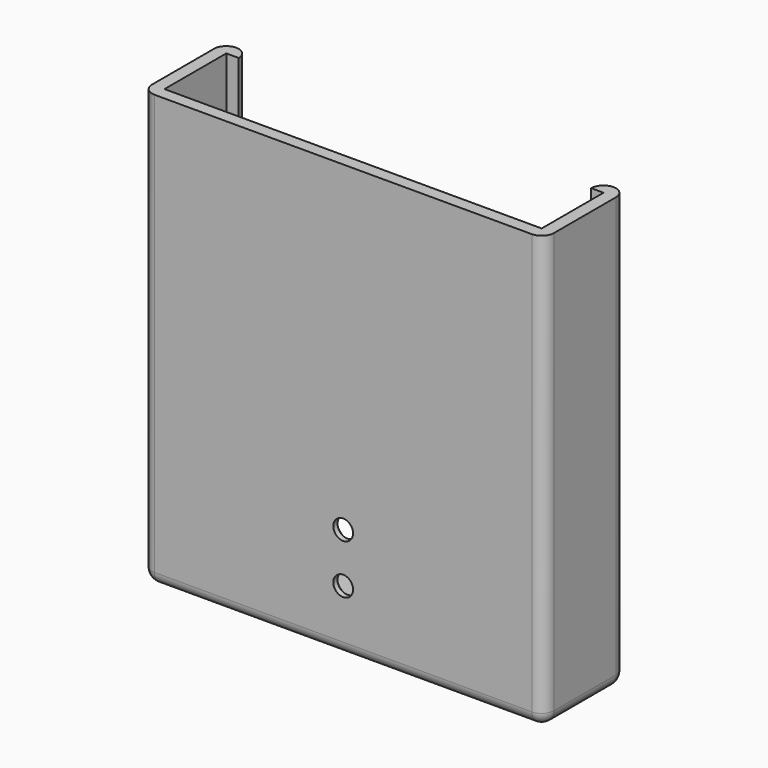
from build123d import *

# Parameters (mm, degrees)
F0_DEPTH       = 70
F1_W           = 65
F1_H           = 16.5
F8_DEPTH       = 2
F2_T1_DEPTH    = 12.5
F2_T3_DEPTH    = 73
F2_T5_DEPTH    = 57
F2_T7_DEPTH    = 61
F2_S11_W       = 2.04
F2_S11_H       = 2.04
F2_T12_DEPTH   = 2.04
F2_S17_W       = 2.04
F2_S17_H       = 2.04
F2_T18_DEPTH   = 2.04
F2_S23_W       = 2.04
F2_S23_H       = 2.04
F2_T24_DEPTH   = 2.04
F2_S29_W       = 2.04
F2_S29_H       = 2.04
F2_T30_DEPTH   = 2.04
F2_T37_DEPTH   = 73
F2_T42_DEPTH   = 62
F2_T50_DEPTH   = 62
F2_T55_DEPTH   = 73
F2_T62_DEPTH   = 17.5
F2_T67_DEPTH   = 17.5
F5_D           = 3.2
F5_CSINK_D     = 5.5
F5_CSINK_ANGLE = 90
F6_D           = 3.2
F6_CSINK_D     = 5.5
F6_CSINK_ANGLE = 90


# Not quite as in the source:
# - a fillet or chamfer that OpenCascade refuses, or shapes differently, is made with other operations: its cross-section is extruded or revolved along the edge and cut away or added
# - a feature names something its author has since deleted; it is built from what else it names


with BuildPart() as f0:
    # F7 (on Top) → F0 (new body)
    with BuildSketch(Plane.XY):
        Polygon((-32.5, 16.5), (-32.5, 0), (32.5, 0), (32.5, 16.5), (28.5, 16.5), (28.5, 14.5), (30.5, 14.5), (30.5, 2), (-30.5, 2), (-30.5, 14.5), (-28.5, 14.5), (-28.5, 16.5), align=None)
    extrude(amount=F0_DEPTH)

    # F1 (on face) → F8 (join)
    with BuildSketch(Plane(origin=(0, 0, 0), x_dir=(1, 0, 0), z_dir=(0, 0, -1))):
        with Locations((0, -8.25)):
            Rectangle(F1_W, F1_H)
    extrude(amount=-F8_DEPTH)

    # F2: fillet of radius 2 on 13 edges, made by hand

    # F2_s2 → F2_t1 (cut)
    with BuildSketch(Plane.XZ.offset(-14.5)):
        with BuildLine():
            ThreePointArc((32.5, 2), (31.9142135624, 0.5857864376), (30.5, 0))
            Line((30.5, 0), (32.5, 0))
            Line((32.5, 0), (32.5, 2))
        make_face()
        with BuildLine():
            ThreePointArc((-32.5, 2), (-31.9142135624, 0.5857864376), (-30.5, 0))
            Line((-30.5, 0), (-32.5, 0))
            Line((-32.5, 0), (-32.5, 2))
        make_face()
    extrude(amount=F2_T1_DEPTH, mode=Mode.SUBTRACT)

    # F2_s4 → F2_t3 (cut)
    with BuildSketch(Plane.XY.offset(2)):
        with BuildLine():
            ThreePointArc((-32.5, 2), (-31.9142135624, 0.5857864376), (-30.5, 0))
            Line((-30.5, 0), (-32.5, 0))
            Line((-32.5, 0), (-32.5, 2))
        make_face()
        with BuildLine():
            ThreePointArc((30.5, 0), (31.9142135624, 0.5857864376), (32.5, 2))
            Line((32.5, 2), (32.5, 0))
            Line((32.5, 0), (30.5, 0))
        make_face()
        with BuildLine():
            ThreePointArc((-32.5, 14.5), (-31.9142135624, 15.9142135624), (-30.5, 16.5))
            Line((-30.5, 16.5), (-32.5, 16.5))
            Line((-32.5, 16.5), (-32.5, 14.5))
        make_face()
        with BuildLine():
            ThreePointArc((32.5, 14.5), (31.9142135624, 15.9142135624), (30.5, 16.5))
            Line((30.5, 16.5), (32.5, 16.5))
            Line((32.5, 16.5), (32.5, 14.5))
        make_face()
        with BuildLine():
            ThreePointArc((-28.5, 14.5), (-29.0857864376, 15.9142135624), (-30.5, 16.5))
            Line((-30.5, 16.5), (-28.5, 16.5))
            Line((-28.5, 16.5), (-28.5, 14.5))
        make_face()
        with BuildLine():
            ThreePointArc((28.5, 14.5), (29.0857864376, 15.9142135624), (30.5, 16.5))
            Line((30.5, 16.5), (28.5, 16.5))
            Line((28.5, 16.5), (28.5, 14.5))
        make_face()
    extrude(amount=F2_T3_DEPTH, mode=Mode.SUBTRACT)

    # F2_s6 → F2_t5 (cut)
    with BuildSketch(Plane.YZ.offset(-28.5)):
        with BuildLine():
            ThreePointArc((14.5, 2), (15.9142135624, 1.4142135624), (16.5, 0))
            Line((16.5, 0), (16.5, 2))
            Line((16.5, 2), (14.5, 2))
        make_face()
    extrude(amount=F2_T5_DEPTH, mode=Mode.SUBTRACT)

    # F2_s8 → F2_t7 (cut)
    with BuildSketch(Plane.YZ.offset(-30.5)):
        with BuildLine():
            ThreePointArc((0, 2), (0.5857864376, 0.5857864376), (2, 0))
            Line((2, 0), (0, 0))
            Line((0, 0), (0, 2))
        make_face()
        with BuildLine():
            ThreePointArc((16.5, 2), (15.9142135624, 0.5857864376), (14.5, 0))
            Line((14.5, 0), (16.5, 0))
            Line((16.5, 0), (16.5, 2))
        make_face()
    extrude(amount=F2_T7_DEPTH, mode=Mode.SUBTRACT)


with BuildPart() as f2_tool10:
    # F2_s11 → F2_t12 (new body)
    with BuildSketch(Plane.XZ.offset(-2)):
        with Locations((31.52, 0.98)):
            Rectangle(F2_S11_W, F2_S11_H)
    extrude(amount=F2_T12_DEPTH)

    # F2_s13 → F2_t14 (revolve, cut)
    with BuildSketch(Plane(origin=(30.5, 2, 2), x_dir=(-0.7071067812, 0, 0.7071067812), z_dir=(0.7071067812, 0, 0.7071067812))):
        with BuildLine():
            ThreePointArc((0, -2), (2, 0), (0, 2))
            Line((0, 2), (0, -2))
        make_face()
    revolve(axis=Axis((30.5, 2, 2), (0, -1, 0)), mode=Mode.SUBTRACT)


with BuildPart() as f0_1:
    add(f0.part)

    # F2_t9: cut F2_tool10
    add(f2_tool10.part, mode=Mode.SUBTRACT)


with BuildPart() as f2_tool16:
    # F2_s17 → F2_t18 (new body)
    with BuildSketch(Plane.YZ.offset(30.5)):
        with Locations((15.52, 0.98)):
            Rectangle(F2_S17_W, F2_S17_H)
    extrude(amount=F2_T18_DEPTH)

    # F2_s19 → F2_t20 (revolve, cut)
    with BuildSketch(Plane(origin=(30.5, 14.5, 2), x_dir=(0, -0.7071067812, 0.7071067812), z_dir=(0, 0.7071067812, 0.7071067812))):
        with BuildLine():
            ThreePointArc((0, -2), (2, 0), (0, 2))
            Line((0, 2), (0, -2))
        make_face()
    revolve(axis=Axis((30.5, 14.5, 2), (1, 0, 0)), mode=Mode.SUBTRACT)


with BuildPart() as f0_2:
    add(f0_1.part)

    # F2_t15: cut F2_tool16
    add(f2_tool16.part, mode=Mode.SUBTRACT)


with BuildPart() as f2_tool22:
    # F2_s23 → F2_t24 (new body)
    with BuildSketch(Plane.YZ.offset(-30.5)):
        with Locations((15.52, 0.98)):
            Rectangle(F2_S23_W, F2_S23_H)
    extrude(amount=-F2_T24_DEPTH)

    # F2_s25 → F2_t26 (revolve, cut)
    with BuildSketch(Plane(origin=(-30.5, 14.5, 2), x_dir=(0, -0.7071067812, 0.7071067812), z_dir=(0, -0.7071067812, -0.7071067812))):
        with BuildLine():
            ThreePointArc((0, -2), (2, 0), (0, 2))
            Line((0, 2), (0, -2))
        make_face()
    revolve(axis=Axis((-30.5, 14.5, 2), (-1, 0, 0)), mode=Mode.SUBTRACT)


with BuildPart() as f0_3:
    add(f0_2.part)

    # F2_t21: cut F2_tool22
    add(f2_tool22.part, mode=Mode.SUBTRACT)


with BuildPart() as f2_tool28:
    # F2_s29 → F2_t30 (new body)
    with BuildSketch(Plane.YZ.offset(-30.5)):
        with Locations((0.98, 0.98)):
            Rectangle(F2_S29_W, F2_S29_H)
    extrude(amount=-F2_T30_DEPTH)

    # F2_s31 → F2_t32 (revolve, cut)
    with BuildSketch(Plane(origin=(-30.5, 2, 2), x_dir=(0, 0.7071067812, 0.7071067812), z_dir=(0, -0.7071067812, 0.7071067812))):
        with BuildLine():
            ThreePointArc((0, -2), (2, 0), (0, 2))
            Line((0, 2), (0, -2))
        make_face()
    revolve(axis=Axis((-30.5, 2, 2), (-1, 0, 0)), mode=Mode.SUBTRACT)


with BuildPart() as f0_4:
    add(f0_3.part)

    # F2_t27: cut F2_tool28
    add(f2_tool28.part, mode=Mode.SUBTRACT)


with BuildPart() as f2_tool35:
    # F2_s36 → F2_t37 (new body)
    with BuildSketch(Plane.XY.offset(-3)):
        with BuildLine():
            ThreePointArc((-28.5, 14.5), (-29.0857864376, 15.9142135624), (-30.5, 16.5))
            Line((-30.5, 16.5), (-28.5, 16.5))
            Line((-28.5, 16.5), (-28.5, 14.5))
        make_face()
    extrude(amount=F2_T37_DEPTH)

    split(bisect_by=Plane.XY.offset(2), keep=Keep.BOTTOM)

    split(bisect_by=Plane.XY, keep=Keep.TOP)


with BuildPart() as f2_tool40:
    # F2_s41 → F2_t42 (new body)
    with BuildSketch(Plane.YZ.offset(-33.5)):
        with BuildLine():
            ThreePointArc((14.5, 2), (15.9142135624, 1.4142135624), (16.5, 0))
            Line((16.5, 0), (16.5, 2))
            Line((16.5, 2), (14.5, 2))
        make_face()
    extrude(amount=F2_T42_DEPTH)

    split(bisect_by=Plane.YZ.offset(-28.5), keep=Keep.BOTTOM)

    split(bisect_by=Plane.YZ.offset(-30.5), keep=Keep.TOP)


with BuildPart() as f2_tool35_1:
    add(f2_tool35.part)

    # F2_t45: intersect F2_tool40
    add(f2_tool40.part, mode=Mode.INTERSECT)


with BuildPart() as f0_5:
    add(f0_4.part)

    # F2_t33: cut F2_tool35
    add(f2_tool35_1.part, mode=Mode.SUBTRACT)


with BuildPart() as f2_tool48:
    # F2_s49 → F2_t50 (new body)
    with BuildSketch(Plane.YZ.offset(-28.5)):
        with BuildLine():
            ThreePointArc((14.5, 2), (15.9142135624, 1.4142135624), (16.5, 0))
            Line((16.5, 0), (16.5, 2))
            Line((16.5, 2), (14.5, 2))
        make_face()
    extrude(amount=F2_T50_DEPTH)

    split(bisect_by=Plane.YZ.offset(30.5), keep=Keep.BOTTOM)

    split(bisect_by=Plane.YZ.offset(28.5), keep=Keep.TOP)


with BuildPart() as f2_tool53:
    # F2_s54 → F2_t55 (new body)
    with BuildSketch(Plane.XY.offset(-3)):
        with BuildLine():
            ThreePointArc((28.5, 14.5), (29.0857864376, 15.9142135624), (30.5, 16.5))
            Line((30.5, 16.5), (28.5, 16.5))
            Line((28.5, 16.5), (28.5, 14.5))
        make_face()
    extrude(amount=F2_T55_DEPTH)

    split(bisect_by=Plane.XY.offset(2), keep=Keep.BOTTOM)

    split(bisect_by=Plane.XY, keep=Keep.TOP)


with BuildPart() as f2_tool48_1:
    add(f2_tool48.part)

    # F2_t58: intersect F2_tool53
    add(f2_tool53.part, mode=Mode.INTERSECT)


with BuildPart() as f0_6:
    add(f0_5.part)

    # F2_t46: cut F2_tool48
    add(f2_tool48_1.part, mode=Mode.SUBTRACT)


with BuildPart() as f2_tool60:
    # F2_s61 → F2_t62 (new body)
    with BuildSketch(Plane.XZ.offset(3)):
        with BuildLine():
            ThreePointArc((30.5, 4), (29.9142135624, 2.5857864376), (28.5, 2))
            Line((28.5, 2), (30.5, 2))
            Line((30.5, 2), (30.5, 4))
        make_face()
    extrude(amount=-F2_T62_DEPTH)

    split(bisect_by=Plane.XZ, keep=Keep.BOTTOM)


with BuildPart() as f0_7:
    add(f0_6.part)

    # F2_t59: union F2_tool60
    add(f2_tool60.part)


with BuildPart() as f2_tool65:
    # F2_s66 → F2_t67 (new body)
    with BuildSketch(Plane.XZ.offset(-14.5)):
        with BuildLine():
            ThreePointArc((-30.5, 4), (-29.9142135624, 2.5857864376), (-28.5, 2))
            Line((-28.5, 2), (-30.5, 2))
            Line((-30.5, 2), (-30.5, 4))
        make_face()
    extrude(amount=F2_T67_DEPTH)

    split(bisect_by=Plane.XZ, keep=Keep.BOTTOM)


with BuildPart() as f0_8:
    add(f0_7.part)

    # F2_t64: union F2_tool65
    add(f2_tool65.part)

    # F5 (through all)
    with Locations(Plane(origin=(0, 2, 0), x_dir=(-1, 0, 0), z_dir=(0, 1, 0))):
        with Locations((0, 18)):
            CounterSinkHole(F5_D / 2, F5_CSINK_D / 2, counter_sink_angle=F5_CSINK_ANGLE)

    # F6 (through all)
    with Locations(Plane(origin=(0, 2, 0), x_dir=(-1, 0, 0), z_dir=(0, 1, 0))):
        with Locations((0, 10)):
            CounterSinkHole(F6_D / 2, F6_CSINK_D / 2, counter_sink_angle=F6_CSINK_ANGLE)


solid = f0_8.part
